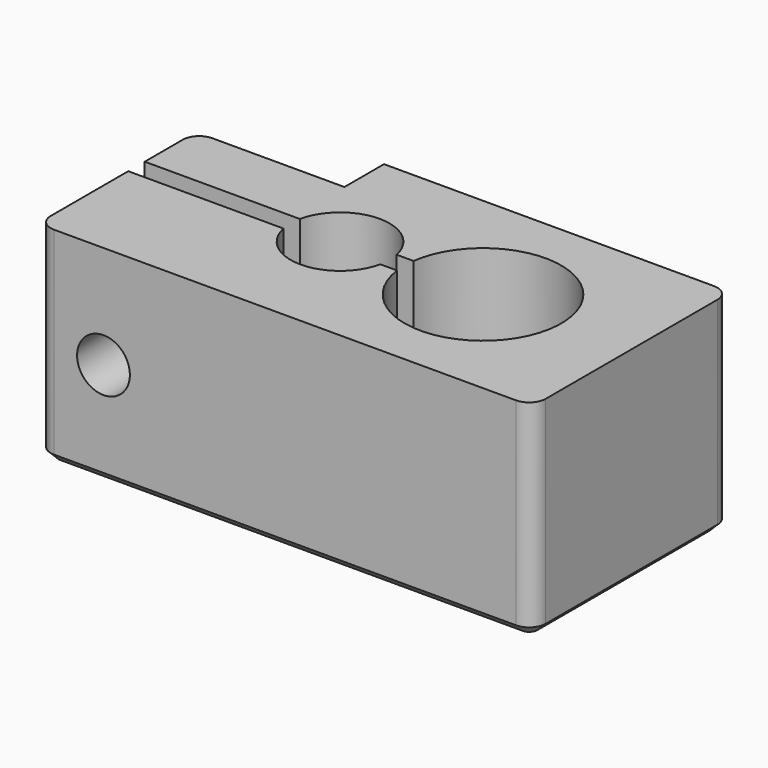
from build123d import *

# Parameters (mm, degrees)
F1_DEPTH = 15
F2_DEPTH = 25
F3_DEPTH = 25
F4_R     = 4
F5_DEPTH = 9
F6_R     = 3.2
F7_DEPTH = 13.5
F8_R     = 2
F9_SIZE  = 1


# Not quite as in the source:
# - a feature names something its author has since deleted; it is built from what else it names


with BuildPart() as f1:
    # F0 (on Top) → F1 (new body)
    with BuildSketch(Plane.XY):
        with BuildLine():
            Line((-30, -1.25), (-30, -15))
            Line((-30, -15), (30, -15))
            Line((30, -15), (30, 15))
            Line((30, 15), (-12, 15))
            Line((-12, 15), (-12, 9))
            Line((-12, 9), (-30, 9))
            Line((-30, 9), (-30, 1.25))
            Line((-30, 1.25), (-11.1936553667, 1.25))
            ThreePointArc((-11.1936553667, 1.25), (-5.3253080696, 6), (0.5430392276, 1.25))
            Line((0.5430392276, 1.25), (2.5825958991, 1.25))
            ThreePointArc((2.5825958991, 1.25), (21.5, 0), (2.5825958991, -1.25))
            Line((2.5825958991, -1.25), (0.5430392276, -1.25))
            ThreePointArc((0.5430392276, -1.25), (-5.3253080696, -6), (-11.1936553667, -1.25))
            Line((-11.1936553667, -1.25), (-30, -1.25))
        make_face()
    extrude(amount=F1_DEPTH)

    # F0 (on Top) + F1_face (on face) → F2 (join)
    with BuildSketch(Plane.XY):
        with BuildLine():
            Line((-30, -1.25), (-30, -15))
            Line((-30, -15), (30, -15))
            Line((30, -15), (30, 15))
            Line((30, 15), (-12, 15))
            Line((-12, 15), (-12, 9))
            Line((-12, 9), (-30, 9))
            Line((-30, 9), (-30, 1.25))
            Line((-30, 1.25), (-11.1936553667, 1.25))
            ThreePointArc((-11.1936553667, 1.25), (-5.3253080696, 6), (0.5430392276, 1.25))
            Line((0.5430392276, 1.25), (2.5825958991, 1.25))
            ThreePointArc((2.5825958991, 1.25), (21.5, 0), (2.5825958991, -1.25))
            Line((2.5825958991, -1.25), (0.5430392276, -1.25))
            ThreePointArc((0.5430392276, -1.25), (-5.3253080696, -6), (-11.1936553667, -1.25))
            Line((-11.1936553667, -1.25), (-30, -1.25))
        make_face()
    with BuildSketch(Plane(origin=(0.3427711831, -1.0419373609, 0), x_dir=(1, 0, 0), z_dir=(0, 0, -1))):
        with BuildLine():
            ThreePointArc((2.239824716, 0.2080626391), (21.1572288169, -1.0419373609), (2.239824716, -2.2919373609))
            Line((2.239824716, -2.2919373609), (0.2002680445, -2.2919373609))
            ThreePointArc((0.2002680445, -2.2919373609), (-5.6680792527, -7.0419373609), (-11.5364265498, -2.2919373609))
            Line((-11.5364265498, -2.2919373609), (-30.3427711831, -2.2919373609))
            Line((-30.3427711831, -2.2919373609), (-30.3427711831, -10.0419373609))
            Line((-30.3427711831, -10.0419373609), (-12.3427711831, -10.0419373609))
            Line((-12.3427711831, -10.0419373609), (-12.3427711831, -16.0419373609))
            Line((-12.3427711831, -16.0419373609), (29.6572288169, -16.0419373609))
            Line((29.6572288169, -16.0419373609), (29.6572288169, 13.9580626391))
            Line((29.6572288169, 13.9580626391), (-30.3427711831, 13.9580626391))
            Line((-30.3427711831, 13.9580626391), (-30.3427711831, 0.2080626391))
            Line((-30.3427711831, 0.2080626391), (-11.5364265498, 0.2080626391))
            ThreePointArc((-11.5364265498, 0.2080626391), (-5.6680792527, 4.9580626391), (0.2002680445, 0.2080626391))
            Line((0.2002680445, 0.2080626391), (2.239824716, 0.2080626391))
        make_face()
    extrude(amount=F2_DEPTH, dir=(0, 0, 1))

    # F0 (on Top) → F3 (join)
    with BuildSketch(Plane.XY):
        with BuildLine():
            Line((-30, -1.25), (-30, -15))
            Line((-30, -15), (30, -15))
            Line((30, -15), (30, 15))
            Line((30, 15), (-12, 15))
            Line((-12, 15), (-12, 9))
            Line((-12, 9), (-30, 9))
            Line((-30, 9), (-30, 1.25))
            Line((-30, 1.25), (-11.1936553667, 1.25))
            ThreePointArc((-11.1936553667, 1.25), (-5.3253080696, 6), (0.5430392276, 1.25))
            Line((0.5430392276, 1.25), (2.5825958991, 1.25))
            ThreePointArc((2.5825958991, 1.25), (21.5, 0), (2.5825958991, -1.25))
            Line((2.5825958991, -1.25), (0.5430392276, -1.25))
            ThreePointArc((0.5430392276, -1.25), (-5.3253080696, -6), (-11.1936553667, -1.25))
            Line((-11.1936553667, -1.25), (-30, -1.25))
        make_face()
    extrude(amount=F3_DEPTH)

    # F4 (on face) → F5 (cut)
    with BuildSketch(Plane(origin=(0, 9, 0), x_dir=(-1, 0, 0), z_dir=(0, 1, 0))):
        with Locations((22, 12.5)):
            Circle(F4_R)
    extrude(amount=-F5_DEPTH, mode=Mode.SUBTRACT)

    # F6 (on face) → F7 (cut)
    with BuildSketch(Plane.XZ.offset(15)):
        with Locations((-22, 12.5)):
            Circle(F6_R)
    extrude(amount=-F7_DEPTH, mode=Mode.SUBTRACT)

    # F8
    f8_edges = [f1.edges().sort_by_distance(p)[0] for p in [
        (30, -15, 12.5),
        (30, 15, 12.5),
        (-30, -15, 12.5),
        (-30, 9, 12.5),
    ]]
    fillet(f8_edges, radius=F8_R)

    # F9
    f9_edges = [f1.edges().sort_by_distance(p)[0] for p in [
        (-30, -7.125, 0),
        (-29.414214, -14.414214, 0),
        (-20.596828, -1.25, 0),
        (0, -15, 0),
        (-5.325308, -6, 0),
        (29.414214, -14.414214, 0),
        (1.562818, -1.25, 0),
        (30, 0, 0),
        (21.5, 0, 0),
        (29.414214, 14.414214, 0),
        (1.562818, 1.25, 0),
        (8, 15, 0),
        (-5.325308, 6, 0),
        (-12, 12, 0),
        (-20.596828, 1.25, 0),
        (-20, 9, 0),
        (-30, 4.125, 0),
        (-29.414214, 8.414214, 0),
    ]]
    chamfer(f9_edges, length=F9_SIZE)


solid = f1.part
